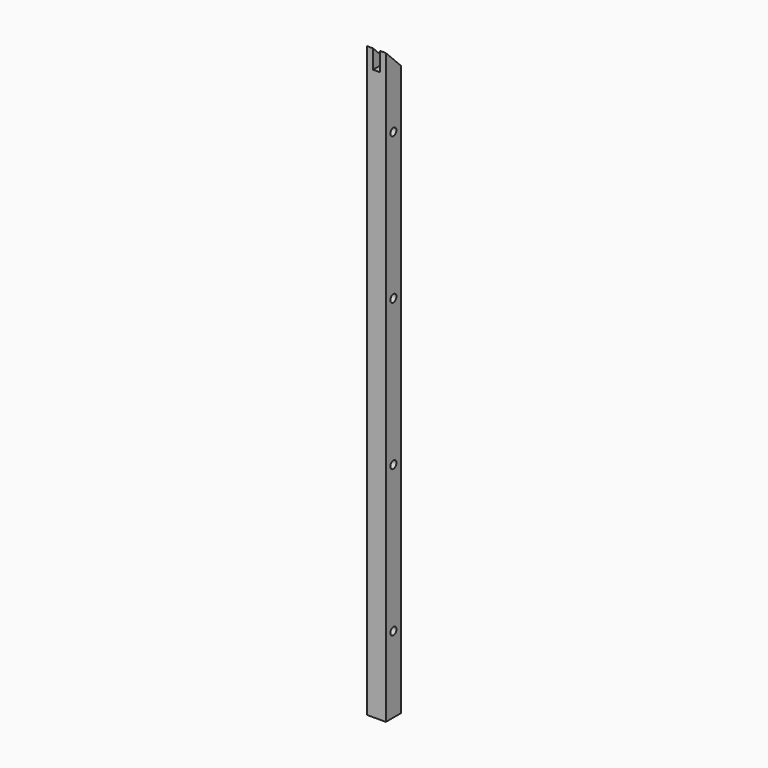
from build123d import *

# Parameters (mm, degrees)
F0_W     = 45
F0_H     = 1407
F1_DEPTH = 22.5
F3_SIZE2 = 44.99999
F3_SIZE  = 44.99999
F2_W     = 16.4
F2_H     = 45
F4_DEPTH = 45
F5_R     = 9
F6_DEPTH = 45.001
F7_DEPTH = 15
F9_D     = 3.5
F9_DEPTH = 30
F9_TIP   = 1.0515060833


# Not quite as in the source:
# - a fillet or chamfer is up to 0.001 mm smaller than in the source, because OpenCascade refuses the exact size


with BuildPart() as f1:
    # F0 (on Front) → F1 (new body, symmetric)
    with BuildSketch(Plane.XZ):
        with Locations((0, -490.1653682211)):
            Rectangle(F0_W, F0_H)
    extrude(amount=F1_DEPTH, both=True)

    # F3 (size 45 and 45 in the source; OpenCascade refuses exactly that, so slightly less here)
    f3_edges = [f1.edges().sort_by_distance(p)[0] for p in [
        (0, 22.5, 213.334632),
    ]]
    chamfer(f3_edges, length=F3_SIZE, length2=F3_SIZE2)

    # F2 (on face) → F4 (cut)
    with BuildSketch(Plane.XY.offset(213.3346317789)):
        Rectangle(F2_W, F2_H)
    extrude(amount=-F4_DEPTH, mode=Mode.SUBTRACT)

    # F5 (on face) → F6 (cut, through all)
    with BuildSketch(Plane(origin=(-22.5, 0, 0), x_dir=(0, -1, 0), z_dir=(-1, 0, 0))):
        with Locations((0, 38.3346317789)):
            Circle(F5_R)
        with Locations((0, -311.6653682211)):
            Circle(F5_R)
        with Locations((0, -661.6653682211)):
            Circle(F5_R)
        with Locations((0, -1011.6653682211)):
            Circle(F5_R)
    extrude(amount=-F6_DEPTH, mode=Mode.SUBTRACT)

    # F5 (on face) → F7 (join)
    with BuildSketch(Plane(origin=(-22.5, 0, 0), x_dir=(0, -1, 0), z_dir=(-1, 0, 0))):
        with Locations((0, -1011.6653682211)):
            Circle(F5_R)
        with Locations((0, -661.6653682211)):
            Circle(F5_R)
        with Locations((0, -311.6653682211)):
            Circle(F5_R)
        with Locations((0, 38.3346317789)):
            Circle(F5_R)
    extrude(amount=-F7_DEPTH)

    # F9
    with Locations(Plane(origin=(0, 22.5, 0), x_dir=(-1, 0, 0), z_dir=(0, 1, 0))):
        with Locations((10, 143.3346317789), (10, 103.3346317789), (10, 63.3346317789), (-10, 63.3346317789), (-10, 103.3346317789), (-10, 143.3346317789)):
            Hole(F9_D / 2, depth=F9_DEPTH)
            with Locations((0, 0, -(F9_DEPTH + F9_TIP / 2))):  # 118° drill point
                Cone(0, F9_D / 2, F9_TIP, mode=Mode.SUBTRACT)


solid = f1.part
